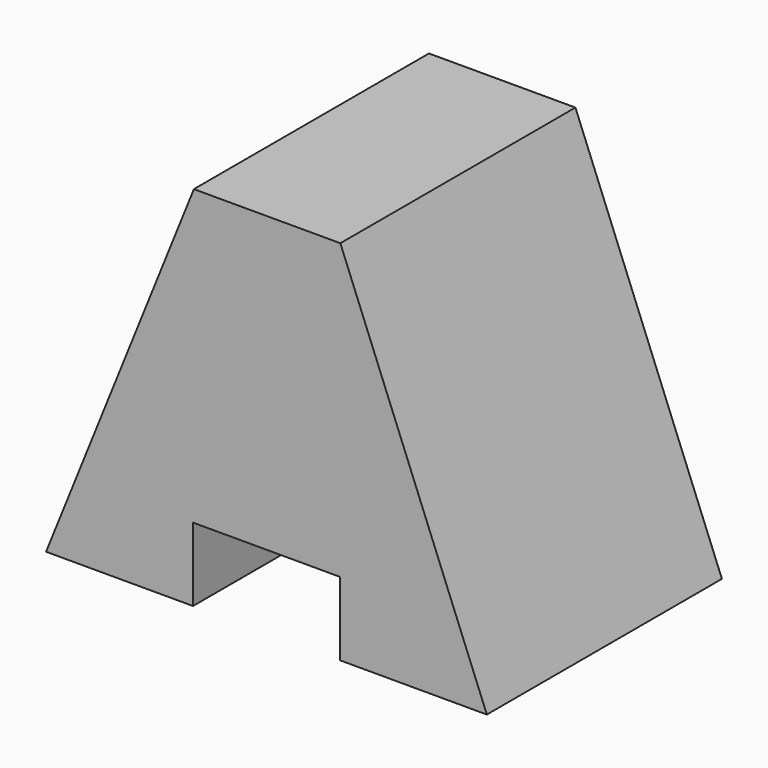
from build123d import *

# Parameters (mm, degrees)
F0_W      = 38.1
F0_H      = 31.75
F2_DEPTH  = 25.4
F7_W      = 12.7
F7_H      = 6.35
F8_DEPTH  = 25.4
F10_DEPTH = 25.4
F12_DEPTH = 25.4


# Not quite as in the source:
# - the program builds the solid bodies; features that only make, move or delete a surface that nothing else refers to are left out


with BuildPart() as f2:
    # F0 (on Front) → F2 (new body)
    with BuildSketch(Plane.XZ):
        with Locations((19.05, 15.875)):
            Rectangle(F0_W, F0_H)
    extrude(amount=F2_DEPTH)

    # F7 (on face) → F8 (cut)
    with BuildSketch(Plane.XZ.offset(25.4)):
        with Locations((19.05, 3.175)):
            Rectangle(F7_W, F7_H)
    extrude(amount=-F8_DEPTH, mode=Mode.SUBTRACT)

    # F9 (on face) → F10 (cut)
    with BuildSketch(Plane.XZ.offset(25.4)):
        Polygon((0, 31.75), (0, 0), (12.7748493105, 31.75), align=None)
    extrude(amount=-F10_DEPTH, mode=Mode.SUBTRACT)

    # F11 (on face) → F12 (cut)
    with BuildSketch(Plane.XZ.offset(25.4)):
        Polygon((25.4374246553, 31.75), (38.1, 0), (38.1, 31.75), align=None)
    extrude(amount=-F12_DEPTH, mode=Mode.SUBTRACT)


solid = f2.part
